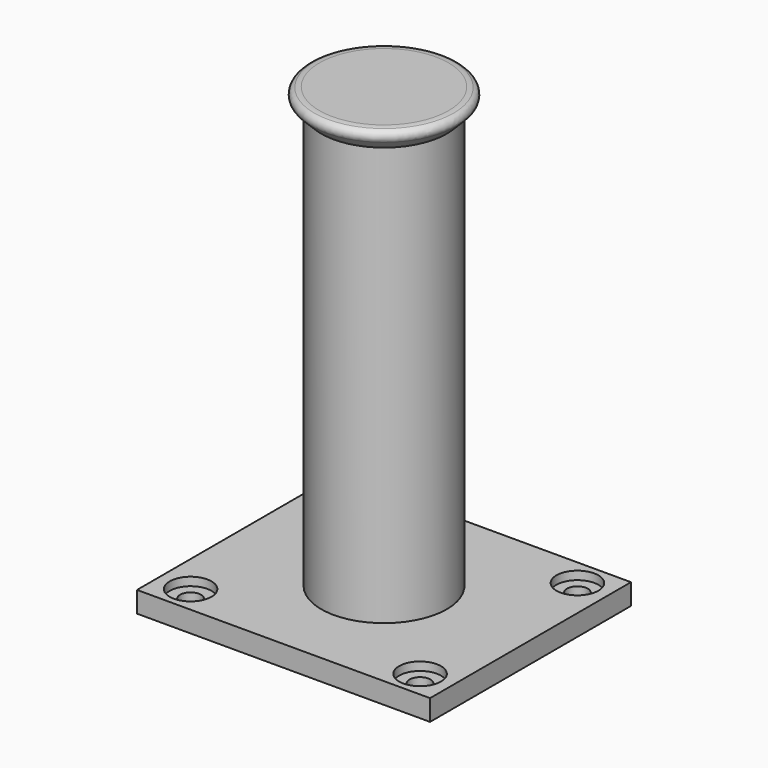
from build123d import *

# Parameters (mm, degrees)
F0_W           = 70
F0_H           = 60
F0_R           = 15
F1_DEPTH       = 5
F2_DEPTH       = 105
F3_R           = 18.75
F3_R_2         = 15
F4_DEPTH       = 5
F5_SIZE        = 3.74999
F7_R           = 1.5
F9_D           = 5
F9_DEPTH       = 5
F9_CBORE_D     = 10
F9_CBORE_DEPTH = 2
F9_TIP         = 1.5021515476


# Not quite as in the source:
# - a fillet or chamfer that OpenCascade refuses, or shapes differently, is made with other operations: its cross-section is extruded or revolved along the edge and cut away or added
# - a fillet or chamfer is up to 0.001 mm smaller than in the source, because OpenCascade refuses the exact size


with BuildPart() as f1:
    # F0 (on Top) → F1 (new body)
    with BuildSketch(Plane.XY):
        Rectangle(F0_W, F0_H)
        Circle(F0_R, mode=Mode.SUBTRACT)
    extrude(amount=F1_DEPTH)

    # F0 (on Top) → F2 (join)
    with BuildSketch(Plane.XY):
        Circle(F0_R)
    extrude(amount=F2_DEPTH)

    # F3 (on face) → F4 (join)
    with BuildSketch(Plane.XY.offset(105)):
        Circle(F3_R)
        Circle(F3_R_2, mode=Mode.SUBTRACT)
        Circle(F3_R_2)
    extrude(amount=F4_DEPTH)

    # F5 (size 3.75 in the source; OpenCascade refuses exactly that, so slightly less here)
    f5_edges = [f1.edges().sort_by_distance(p)[0] for p in [
        (-18.75, 0, 105),
    ]]
    chamfer(f5_edges, length=F5_SIZE)

    # F6: fillet of radius 5 on 1 edges, made by hand

    # F6_s1 → F6_t2 (revolve, cut)
    with BuildSketch(Plane.XZ):
        with BuildLine():
            ThreePointArc((18.75, 108.74999), (17.2105735463, 109.6770690609), (15.4427995223, 110))
            Line((15.4427995223, 110), (18.75, 110))
            Line((18.75, 110), (18.75, 108.74999))
        make_face()
    revolve(axis=Axis((0, 0, 110), (0, 0, 1)), mode=Mode.SUBTRACT)

    # F7
    f7_edges = [f1.edges().sort_by_distance(p)[0] for p in [
        (-18.75, 0, 108.74999),
    ]]
    fillet(f7_edges, radius=F7_R)

    # F9
    with Locations(Plane.XY.offset(5)):
        with Locations((-27.4074339763, 23.4920862654), (-27.4074339763, -23.4920862654), (27.4074339763, -23.4920862654), (27.4074339763, 23.4920862654)):
            CounterBoreHole(F9_D / 2, F9_CBORE_D / 2, F9_CBORE_DEPTH, depth=F9_DEPTH)
            with Locations((0, 0, -(F9_DEPTH + F9_TIP / 2))):  # 118° drill point
                Cone(0, F9_D / 2, F9_TIP, mode=Mode.SUBTRACT)


solid = f1.part
